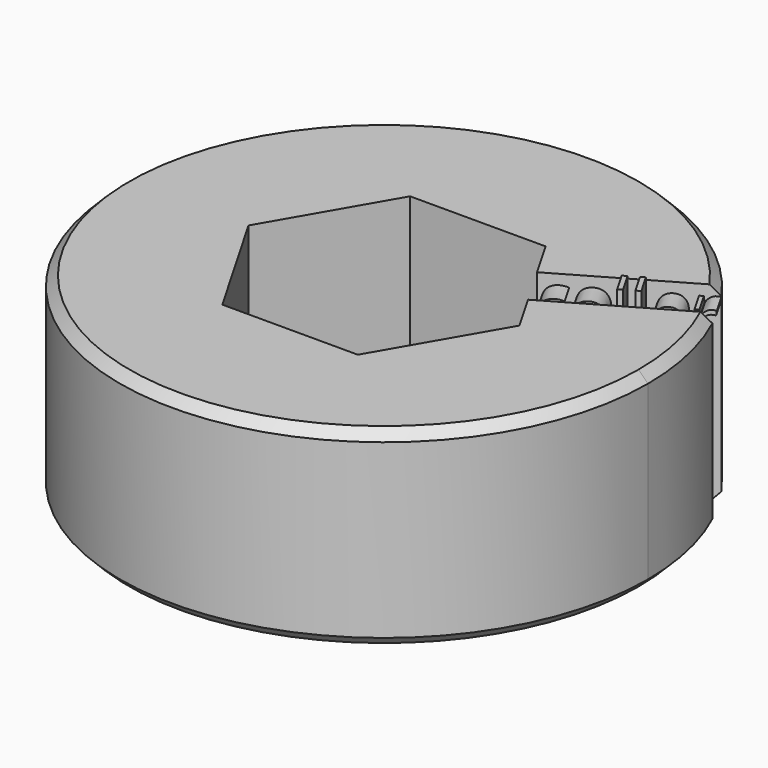
from build123d import *

# Parameters (mm, degrees)
F1_DEPTH     = 10.3378
F2_SIZE      = 0.508
F3_TEXT_SIZE = 3.1012075229
F3_W         = 0.2514885476
F3_H         = 2.2328694165
F4_DEPTH     = 1.27


# Not quite as in the source:
# - Text() gives the source's letters only with a copy of the font that has no kerning and outlines rounded to 1/6400 em; it was checked with that copy


with BuildPart() as f1:
    # F0 (on Top) → F1 (new body)
    with BuildSketch(Plane.XY):
        with BuildLine():
            ThreePointArc((11.6893586927, 8.2153240717), (-12.6789017451, 6.5862057961), (0, -14.2875))
            Line((0, -14.2875), (0, -6.35))
            Line((0, -6.35), (-3.6661742094, -6.35))
            Line((-3.6661742094, -6.35), (-7.3323484187, 0))
            Line((-7.3323484187, 0), (-3.6661742094, 6.35))
            Line((-3.6661742094, 6.35), (3.6661742094, 6.35))
            Line((3.6661742094, 6.35), (4.864261314, 4.2748522628))
            Line((4.864261314, 4.2748522628), (11.6893586927, 8.2153240717))
        make_face()
        with BuildLine():
            Line((0, -6.35), (0, -14.2875))
            ThreePointArc((0, -14.2875), (10.1027881362, -10.1027881362), (14.2875, 0))
            ThreePointArc((14.2875, 0), (13.9515141396, 3.0802450331), (12.9593586927, 6.015619546))
            Line((12.9593586927, 6.015619546), (6.134261314, 2.0751477372))
            Line((6.134261314, 2.0751477372), (7.3323484187, 0))
            Line((7.3323484187, 0), (3.6661742094, -6.35))
            Line((3.6661742094, -6.35), (0, -6.35))
        make_face()
    extrude(amount=F1_DEPTH)

    # F2
    f2_edges = [f1.edges().sort_by_distance(p)[0] for p in [
        (-12.373338, -7.14375, 10.3378),
        (-12.373338, -7.14375, 0),
    ]]
    chamfer(f2_edges, length=F2_SIZE)

    # F3 (on face) → F4 (join)
    with BuildSketch(Plane(origin=(-0.635, 1.0998522628, 0), x_dir=(0.8660254038, 0.5, 0), z_dir=(0.5, -0.8660254038, 0))):
        with Locations((6.35, 8.1049305835)):
            Text('coller', F3_TEXT_SIZE, font='Open Sans', text_align=(TextAlign.LEFT, TextAlign.BOTTOM))
        with Locations((10.8765515743, 9.2213652917)):
            Rectangle(F3_W, F3_H)
    extrude(amount=F4_DEPTH)


solid = f1.part
